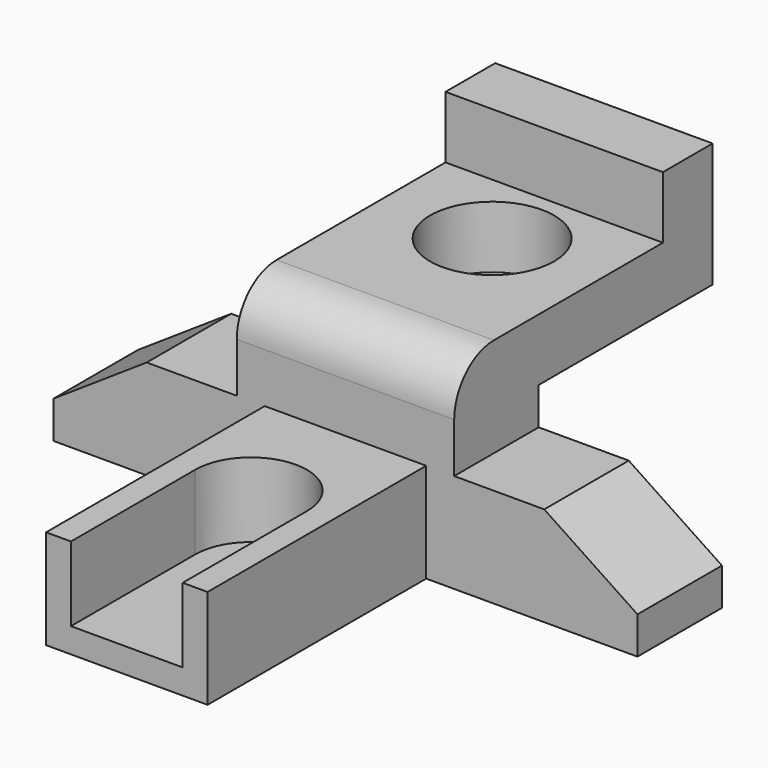
from build123d import *

# Parameters (mm, degrees)
F1_DEPTH  = 17
F2_W      = 26
F2_H      = 16
F3_DEPTH  = 44
F4_W      = 18
F4_H      = 25
F5_DEPTH  = 12
F8_DEPTH  = 17.5
F9_R      = 8
F10_R     = 10
F11_DEPTH = 25


# Not quite as in the source:
# - the program builds the solid bodies; features that only make, move or delete a surface that nothing else refers to are left out


with BuildPart() as f1:
    # F0 (on Front) → F1 (new body)
    with BuildSketch(Plane.XZ):
        Polygon((52.0617456436, 19.5316821036), (37.0617456436, 29.5316821036), (-26.9382543564, 29.5316821036), (-41.9382543564, 19.5316821036), (-41.9382543564, 13.5316821036), (52.0617456436, 13.5316821036), align=None)
    extrude(amount=F1_DEPTH)

    # F2 (on face) → F3 (join)
    with BuildSketch(Plane.XZ.offset(17)):
        with Locations((5.0617456436, 21.5316821036)):
            Rectangle(F2_W, F2_H)
    extrude(amount=F3_DEPTH)

    # F4 (on face) → F5 (cut)
    with BuildSketch(Plane.XY.offset(29.5316821036)):
        with Locations((5.0617456436, -48.5)):
            Rectangle(F4_W, F4_H)
        with BuildLine():
            Line((-3.9382543564, -36), (14.0617456436, -36))
            ThreePointArc((14.0617456436, -36), (5.0617456436, -27), (-3.9382543564, -36))
        make_face()
    extrude(amount=-F5_DEPTH, mode=Mode.SUBTRACT)

    # F7 (on offset) → F8 (join, symmetric)
    with BuildSketch(Plane.YZ.offset(5.0617456436)):
        Polygon((-17, 45.5316821036), (-17, 29.5316821036), (0, 29.5316821036), (0, 35.5316821036), (35, 35.5316821036), (35, 55.5316821036), (25, 55.5316821036), (25, 45.5316821036), align=None)
    extrude(amount=F8_DEPTH, both=True)

    # F9
    f9_edges = [f1.edges().sort_by_distance(p)[0] for p in [
        (5.061746, -17, 45.531682),
    ]]
    fillet(f9_edges, radius=F9_R)

    # F10 (on face) → F11 (cut)
    with BuildSketch(Plane.XY.offset(45.5316821036)):
        with Locations((5.0617456436, 12.5)):
            Circle(F10_R)
    extrude(amount=-F11_DEPTH, mode=Mode.SUBTRACT)


solid = f1.part
